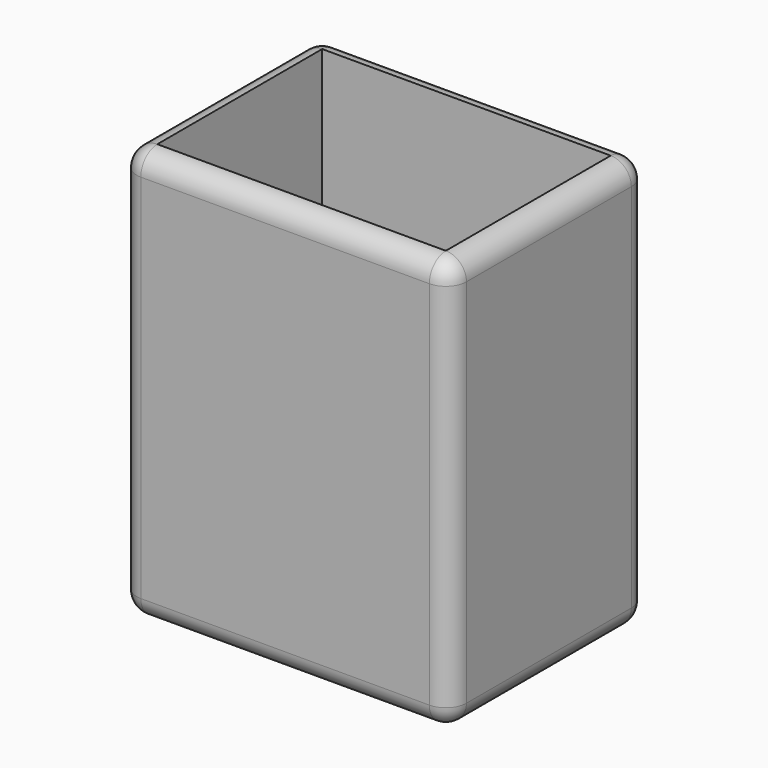
from build123d import *

# Parameters (mm, degrees)
F0_W     = 101.6
F0_H     = 76.2
F1_DEPTH = 127
F2_T     = -6.35
F3_R     = 6.34999


# Not quite as in the source:
# - a fillet or chamfer is up to 0.001 mm smaller than in the source, because OpenCascade refuses the exact size


with BuildPart() as f1:
    # F0 (on Top) → F1 (new body)
    with BuildSketch(Plane.XY):
        with Locations((-6.6963651597, -9.8136370122)):
            Rectangle(F0_W, F0_H)
    extrude(amount=F1_DEPTH)

    # F2
    f2_openings = [f1.faces().sort_by_distance(p)[0] for p in [
        (-6.696365, -9.813637, 127),
    ]]
    offset(amount=F2_T, openings=f2_openings)

    # F3 (radius 6.35 in the source; OpenCascade refuses exactly that, so slightly less here)
    f3_edges = [f1.edges().sort_by_distance(p)[0] for p in [
        (-57.496365, -47.913637, 63.5),
        (-57.496365, 28.286363, 63.5),
        (-57.496365, -9.813637, 0),
        (-57.496365, -9.813637, 127),
        (44.103635, 28.286363, 63.5),
        (-6.696365, 28.286363, 0),
        (-6.696365, 28.286363, 127),
        (44.103635, -47.913637, 63.5),
        (44.103635, -9.813637, 0),
        (44.103635, -9.813637, 127),
        (-6.696365, -47.913637, 0),
        (-6.696365, -47.913637, 127),
    ]]
    fillet(f3_edges, radius=F3_R)


solid = f1.part
